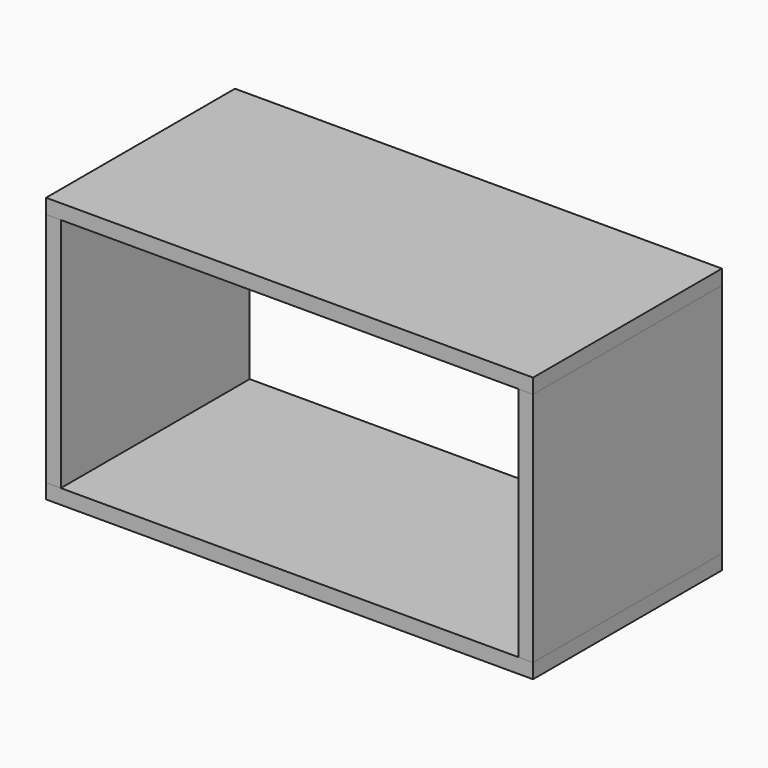
from build123d import *

# Parameters (mm, degrees)
F2_DEPTH      = 50.8
F1_W          = 6.35
F1_H          = 50.8
F3_DEPTH      = 50.8
F3_DEPTH_BACK = 50.8


# Not quite as in the source:
# - a variable given as a bare number and used for a length is read in inches; the dataset says mm whatever the document's units were


with BuildPart() as f2:
    # F1 (on Front) → F2 (new body, symmetric)
    with BuildSketch(Plane.XZ):
        Polygon((104.775, 0), (-104.775, 0), (-104.775, -6.35), (-98.425, -6.35), (98.425, -6.35), (104.775, -6.35), align=None)
    extrude(amount=F2_DEPTH, both=True)


with BuildPart() as f2b:
    # F1 (on Front) → F2, piece 2 (new body, symmetric)
    with BuildSketch(Plane.XZ):
        Polygon((104.775, -114.3), (104.775, -107.95), (98.425, -107.95), (-98.425, -107.95), (-104.775, -107.95), (-104.775, -114.3), align=None)
    extrude(amount=F2_DEPTH, both=True)


with BuildPart() as f3:
    # F1 (on Front) → F3 (new body, two sides)
    with BuildSketch(Plane.XZ) as f3_sk:
        with Locations((-101.6, -31.75)):
            Rectangle(F1_W, F1_H)
        with Locations((-101.6, -82.55)):
            Rectangle(F1_W, F1_H)
    extrude(amount=F3_DEPTH)
    extrude(f3_sk.sketch, amount=-F3_DEPTH_BACK)


with BuildPart() as f3b:
    # F1 (on Front) → F3, piece 2 (new body, two sides)
    with BuildSketch(Plane.XZ) as f3_2_sk:
        Polygon((104.775, -107.95), (104.775, -6.35), (98.425, -6.35), (98.425, -57.15), (98.425, -107.95), align=None)
    extrude(amount=F3_DEPTH)
    extrude(f3_2_sk.sketch, amount=-F3_DEPTH_BACK)


solid = Compound([f2.part, f2b.part, f3.part, f3b.part])
